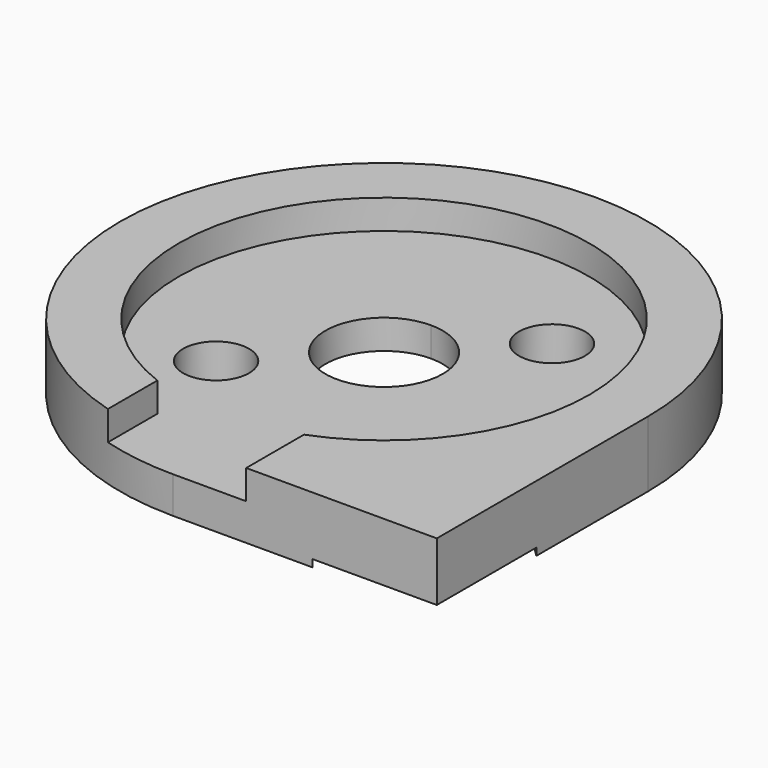
from build123d import *

# Parameters (mm, degrees)
F0_R     = 14
F1_DEPTH = 2
F2_DEPTH = 2.5
F3_DEPTH = 3
F5_DEPTH = 0.5
F7_DEPTH = 2


# Not quite as in the source:
# - a feature names something its author has since deleted; it is built from what else it names


with BuildPart() as f1:
    # F0 (on Top) → F1 (new body)
    with BuildSketch(Plane.XY):
        with BuildLine():
            Line((18, -18), (18, 0))
            ThreePointArc((18, 0), (12.7279220614, 12.7279220614), (0, 18))
            ThreePointArc((0, 18), (-12.7279220614, 12.7279220614), (-18, 0))
            ThreePointArc((-18, 0), (-12.7279220614, -12.7279220614), (0, -18))
            Line((0, -18), (18, -18))
        make_face()
        Circle(F0_R, mode=Mode.SUBTRACT)
    extrude(amount=F1_DEPTH)

    # F0 (on Top) → F2 (join)
    with BuildSketch(Plane.XY):
        with BuildLine():
            Line((18, -18), (18, 0))
            ThreePointArc((18, 0), (12.7279220614, 12.7279220614), (0, 18))
            ThreePointArc((0, 18), (-12.7279220614, 12.7279220614), (-18, 0))
            ThreePointArc((-18, 0), (-12.7279220614, -12.7279220614), (0, -18))
            Line((0, -18), (18, -18))
        make_face()
        Circle(F0_R, mode=Mode.SUBTRACT)
        Circle(F0_R)
        with BuildLine():
            ThreePointArc((-4.1139610307, -6.3639610307), (-8.4426899788, -7.2249987535), (-4.772970773, -4.772970773))
            ThreePointArc((-4.772970773, -4.772970773), (-4.2852320825, -5.5029233079), (-4.1139610307, -6.3639610307))
        make_face(mode=Mode.SUBTRACT)
        with BuildLine():
            ThreePointArc((2.8284271247, 2.8284271247), (3.69551813, 1.5307337295), (4, 0))
            ThreePointArc((4, 0), (1.5307337295, -3.69551813), (-2.8284271247, -2.8284271247))
            ThreePointArc((-2.8284271247, -2.8284271247), (-3.69551813, 1.5307337295), (0, 4))
            ThreePointArc((0, 4), (1.5307337295, 3.69551813), (2.8284271247, 2.8284271247))
        make_face(mode=Mode.SUBTRACT)
        with BuildLine():
            ThreePointArc((8.6139610307, 6.3639610307), (7.2249987535, 4.2852320825), (4.772970773, 4.772970773))
            ThreePointArc((4.772970773, 4.772970773), (5.5029233079, 8.4426899788), (8.6139610307, 6.3639610307))
        make_face(mode=Mode.SUBTRACT)
        with BuildLine():
            ThreePointArc((-2.8284271247, -2.8284271247), (1.5307337295, -3.69551813), (4, 0))
            Line((4, 0), (0, 0))
            Line((0, 0), (-2.8284271247, -2.8284271247))
        make_face()
        with BuildLine():
            Line((0, 0), (2.8284271247, 2.8284271247))
            ThreePointArc((2.8284271247, 2.8284271247), (1.5307337295, 3.69551813), (0, 4))
            Line((0, 4), (0, 0))
        make_face()
        with BuildLine():
            ThreePointArc((0, 4), (-3.69551813, 1.5307337295), (-2.8284271247, -2.8284271247))
            Line((-2.8284271247, -2.8284271247), (0, 0))
            Line((0, 0), (0, 4))
        make_face()
        with BuildLine():
            Line((0, 0), (4, 0))
            ThreePointArc((4, 0), (3.69551813, 1.5307337295), (2.8284271247, 2.8284271247))
            Line((2.8284271247, 2.8284271247), (0, 0))
        make_face()
    extrude(amount=-F2_DEPTH)

    # F0 (on Top) → F3 (cut)
    with BuildSketch(Plane.XY):
        with BuildLine():
            ThreePointArc((-2.8284271247, -2.8284271247), (1.5307337295, -3.69551813), (4, 0))
            Line((4, 0), (0, 0))
            Line((0, 0), (-2.8284271247, -2.8284271247))
        make_face()
        with BuildLine():
            Line((0, 0), (4, 0))
            ThreePointArc((4, 0), (3.69551813, 1.5307337295), (2.8284271247, 2.8284271247))
            Line((2.8284271247, 2.8284271247), (0, 0))
        make_face()
        with BuildLine():
            Line((0, 0), (2.8284271247, 2.8284271247))
            ThreePointArc((2.8284271247, 2.8284271247), (1.5307337295, 3.69551813), (0, 4))
            Line((0, 4), (0, 0))
        make_face()
        with BuildLine():
            ThreePointArc((0, 4), (-3.69551813, 1.5307337295), (-2.8284271247, -2.8284271247))
            Line((-2.8284271247, -2.8284271247), (0, 0))
            Line((0, 0), (0, 4))
        make_face()
    extrude(amount=-F3_DEPTH, mode=Mode.SUBTRACT)

    # F4 (on face) → F5 (cut)
    with BuildSketch(Plane(origin=(0, 0, -2.5), x_dir=(1, 0, 0), z_dir=(0, 0, -1))):
        Polygon((4.2426406871, -4.2426406871), (0, 0), (-4.2426406871, 4.2426406871), (-16.9705627485, -8.4852813742), (-8.4852813742, -16.9705627485), align=None)
        Polygon((8.4852813742, 0), (0, 0), (4.2426406871, -4.2426406871), align=None)
        with BuildLine():
            Line((-2.8284271247, 2.8284271247), (0, 0))
            Line((0, 0), (4, 0))
            ThreePointArc((4, 0), (1.5307337295, 3.69551813), (-2.8284271247, 2.8284271247))
        make_face()
        with BuildLine():
            Line((-4.2426406871, 4.2426406871), (-2.8284271247, 2.8284271247))
            ThreePointArc((-2.8284271247, 2.8284271247), (1.5307337295, 3.69551813), (4, 0))
            Line((4, 0), (8.4852813742, 0))
            Line((8.4852813742, 0), (18, 9.5147186258))
            Line((18, 9.5147186258), (18, 18))
            Line((18, 18), (9.5147186258, 18))
            Line((9.5147186258, 18), (-4.2426406871, 4.2426406871))
        make_face()
    extrude(amount=-F5_DEPTH, mode=Mode.SUBTRACT)

    # F6 (on face) → F7 (cut)
    with BuildSketch(Plane.XY.offset(2)):
        with BuildLine():
            Line((5, -9), (0, -9))
            Line((0, -9), (0, -14))
            ThreePointArc((0, -14), (2.542267135, -13.7672392953), (5, -13.0766968306))
            Line((5, -13.0766968306), (5, -9))
        make_face()
        with BuildLine():
            Line((0, -14), (0, -9))
            Line((0, -9), (-5, -9))
            Line((-5, -9), (-5, -13.0766968306))
            ThreePointArc((-5, -13.0766968306), (-2.542267135, -13.7672392953), (0, -14))
        make_face()
        with BuildLine():
            Line((5, -18), (0, -18))
            ThreePointArc((0, -18), (-2.5249657043, -17.8220242451), (-5, -17.2916164658))
            Line((-5, -17.2916164658), (-5, -19))
            Line((-5, -19), (5, -19))
            Line((5, -19), (5, -18))
        make_face()
        with BuildLine():
            ThreePointArc((5, -13.0766968306), (2.542267135, -13.7672392953), (0, -14))
            Line((0, -14), (0, -18))
            Line((0, -18), (5, -18))
            Line((5, -18), (5, -13.0766968306))
        make_face()
        with BuildLine():
            Line((0, -18), (0, -14))
            ThreePointArc((0, -14), (-2.542267135, -13.7672392953), (-5, -13.0766968306))
            Line((-5, -13.0766968306), (-5, -17.2916164658))
            ThreePointArc((-5, -17.2916164658), (-2.5249657043, -17.8220242451), (0, -18))
        make_face()
    extrude(amount=-F7_DEPTH, mode=Mode.SUBTRACT)


solid = f1.part
